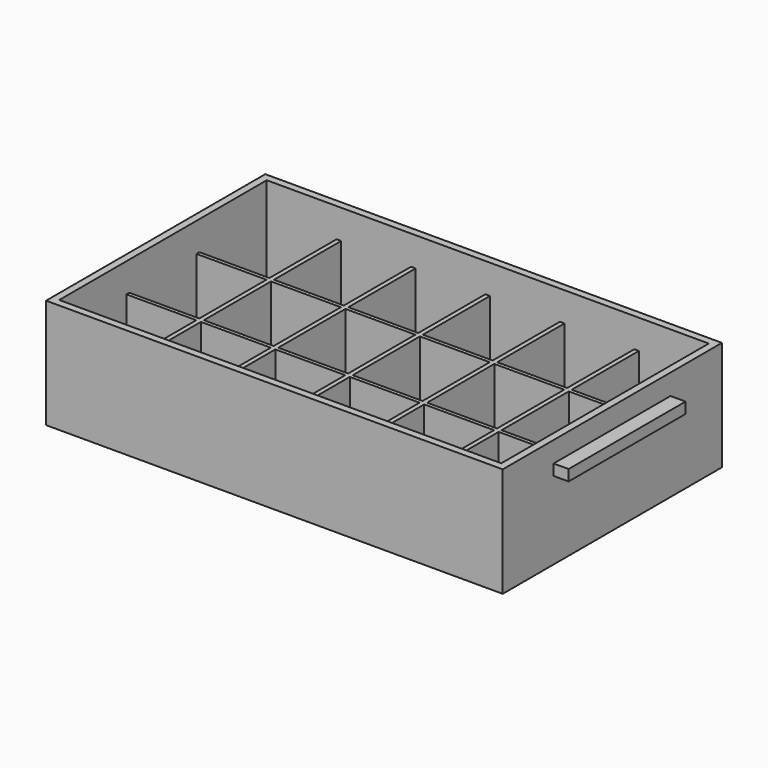
from build123d import *

# Parameters (mm, degrees)
F0_W     = 250
F0_H     = 150
F1_DEPTH = 60
F2_T     = -4
F3_W     = 38.25
F3_H     = 46
F4_DEPTH = 40
F5_W     = 80
F5_H     = 6
F6_DEPTH = 10


# Not quite as in the source:
# - a pattern or mirror of a feature is missing from the dataset's text; its kind, count and spacing are read off the source's solid


with BuildPart() as f1:
    # F0 (on Top) → F1 (new body)
    with BuildSketch(Plane.XY):
        with Locations((0.8881594986, -9.8060739803)):
            Rectangle(F0_W, F0_H)
    extrude(amount=F1_DEPTH)

    # F2
    f2_openings = [f1.faces().sort_by_distance(p)[0] for p in [
        (0.888159, -9.806074, 60),
    ]]
    offset(amount=F2_T, openings=f2_openings)

    # F3 (on face) → F4 (join)
    with BuildSketch(Plane.XY.offset(4)):
        Polygon((-81.8618405014, 15.1939260197), (-120.1118405014, 15.1939260197), (-120.1118405014, 13.1939260197), (-81.8618405014, 13.1939260197), (-81.8618405014, -32.8060739803), (-120.1118405014, -32.8060739803), (-120.1118405014, -34.8060739803), (-81.8618405014, -34.8060739803), (-81.8618405014, -80.8060739803), (-79.3618405014, -80.8060739803), (-79.3618405014, -34.8060739803), (-41.1118405014, -34.8060739803), (-41.1118405014, -80.8060739803), (-38.6118405014, -80.8060739803), (-38.6118405014, -34.8060739803), (-0.3618405014, -34.8060739803), (-0.3618405014, -80.8060739803), (2.1381594986, -80.8060739803), (2.1381594986, -34.8060739803), (40.3881594986, -34.8060739803), (40.3881594986, -80.8060739803), (42.8881594986, -80.8060739803), (42.8881594986, -34.8060739803), (81.1381594986, -34.8060739803), (81.1381594986, -80.8060739803), (83.6381594986, -80.8060739803), (83.6381594986, -34.8060739803), (121.8881594986, -34.8060739803), (121.8881594986, -32.8060739803), (83.6381594986, -32.8060739803), (83.6381594986, 13.1939260197), (121.8881594986, 13.1939260197), (121.8881594986, 15.1939260197), (83.6381594986, 15.1939260197), (83.6381594986, 61.1939260197), (81.1381594986, 61.1939260197), (81.1381594986, 15.1939260197), (42.8881594986, 15.1939260197), (42.8881594986, 61.1939260197), (40.3881594986, 61.1939260197), (40.3881594986, 15.1939260197), (2.1510550287, 15.1939260197), (2.1381594986, 15.1939260197), (2.1381594986, 61.1939260197), (-0.3618405014, 61.1939260197), (-0.3618405014, 15.1939260197), (-38.6118405014, 15.1939260197), (-38.6118405014, 61.1939260197), (-41.1118405014, 61.1939260197), (-41.1118405014, 15.1939260197), (-79.3618405014, 15.1939260197), (-79.3618405014, 61.1939260197), (-81.8618405014, 61.1939260197), align=None)
        with Locations((-60.2368405014, -9.8060739803)):
            Rectangle(F3_W, F3_H, mode=Mode.SUBTRACT)
        with Locations((-19.4868405014, -9.8060739803)):
            Rectangle(F3_W, F3_H, mode=Mode.SUBTRACT)
        with Locations((21.2631594986, -9.8060739803)):
            Rectangle(F3_W, F3_H, mode=Mode.SUBTRACT)
        with Locations((62.0131594986, -9.8060739803)):
            Rectangle(F3_W, F3_H, mode=Mode.SUBTRACT)
    extrude(amount=F4_DEPTH)

    # F5 (on face) → F6 (join)
    with BuildSketch(Plane(origin=(-124.1118405014, 0, 0), x_dir=(0, -1, 0), z_dir=(-1, 0, 0))):
        with Locations((10, 45.6811115146)):
            Rectangle(F5_W, F5_H)
    f6 = extrude(amount=F6_DEPTH)

    # F6_copies: F6 across plane
    add(f6.mirror(Plane(origin=(0, 0, 0), x_dir=(0, 0, 1), z_dir=(1, 0, 0))))


solid = f1.part
